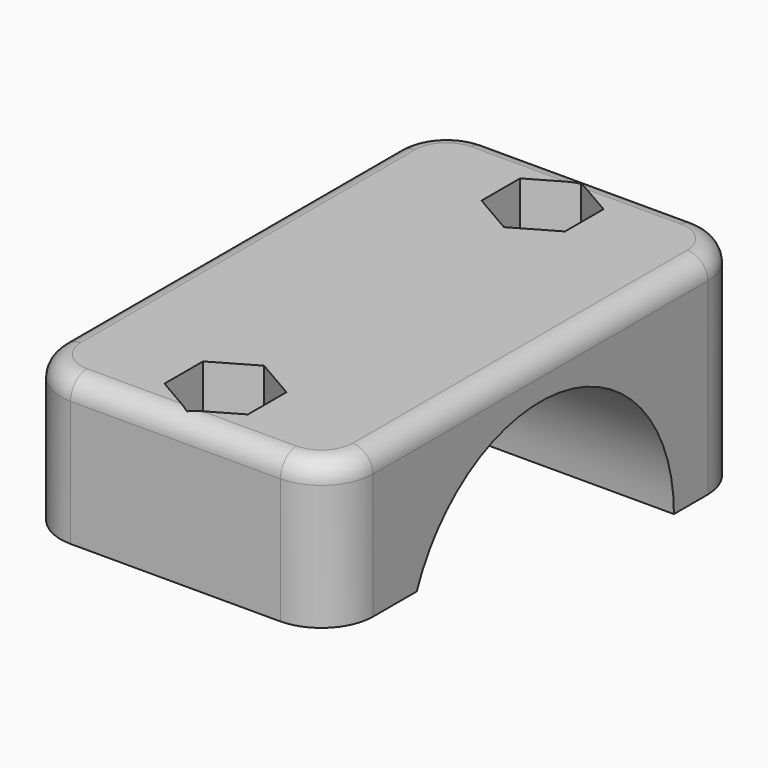
from build123d import *

# Parameters (mm, degrees)
F0_W         = 30
F0_H         = 25
F1_DEPTH     = 20
F3_DEPTH     = 50
F4_D         = 5
F5_R         = 2.5
F6_DEPTH     = 6
F7_T1_DEPTH  = 45.0048285071
F8_T1_DEPTH  = 40.1245744794
F8_T3_DEPTH  = 20.1245744794
F8_T6_ANGLE  = 88.5507069449
F8_T8_ANGLE  = 88.5507069449
F8_T10_ANGLE = 88.550706945
F8_T12_ANGLE = 88.550706945
F9_W         = 14.9377127603
F9_H         = 6
F10_DEPTH    = 50


# Not quite as in the source:
# - a fillet or chamfer that OpenCascade refuses, or shapes differently, is made with other operations: its cross-section is extruded or revolved along the edge and cut away or added


with BuildPart() as f1:
    # F0 (on Top) → F1 (new body)
    with BuildSketch(Plane.XY):
        with Locations((0, 12.5)):
            Rectangle(F0_W, F0_H)
        with Locations((0, -12.5)):
            Rectangle(F0_W, F0_H)
    extrude(amount=F1_DEPTH)

    # F2 (on face) → F3 (cut)
    with BuildSketch(Plane.YZ.offset(15)):
        with BuildLine():
            Line((-16, 0), (16, 0))
            ThreePointArc((16, 0), (0, 16), (-16, 0))
        make_face()
        with BuildLine():
            ThreePointArc((-16, 0), (0, -16), (16, 0))
            Line((16, 0), (-16, 0))
        make_face()
    extrude(amount=-F3_DEPTH, mode=Mode.SUBTRACT)

    # F4 (through all)
    with Locations(Plane(origin=(0, 0, 0), x_dir=(1, 0, 0), z_dir=(0, 0, -1))):
        with Locations((0, -19), (0, 19)):
            Hole(F4_D / 2)

    # F5 (on face) → F6 (cut)
    with BuildSketch(Plane.XY.offset(20)):
        Polygon((4, 16.6905989232), (4, 21.3094010768), (0, 23.6188021535), (-4, 21.3094010768), (-4, 16.6905989232), (0, 14.3811978465), align=None)
        with Locations((0, 19)):
            Circle(F5_R, mode=Mode.SUBTRACT)
        Polygon((4, -21.3094010768), (4, -16.6905989232), (0, -14.3811978465), (-4, -16.6905989232), (-4, -21.3094010768), (0, -23.6188021535), align=None)
        with Locations((0, -19)):
            Circle(F5_R, mode=Mode.SUBTRACT)
    extrude(amount=-F6_DEPTH, mode=Mode.SUBTRACT)

    # F7: fillet of radius 5 on 4 edges, made by hand

    # F7_s2 → F7_t1 (cut)
    with BuildSketch(Plane.XY.offset(-12.5024142536)):
        with BuildLine():
            ThreePointArc((-15.0004, 19.9990343146), (-13.5355339059, 23.5355339059), (-9.9990343146, 25.0004))
            Line((-9.9990343146, 25.0004), (-9.9990343146, 25.5005365685))
            ThreePointArc((-9.9990343146, 25.5005365685), (-12.4995171573, 25.5001365685), (-15, 25.5001365685))
            Line((-15, 25.5001365685), (-15.5001365685, 25))
            ThreePointArc((-15.5001365685, 25), (-15.5001365685, 22.4995171573), (-15.5005365685, 19.9990343146))
            Line((-15.5005365685, 19.9990343146), (-15.0004, 19.9990343146))
        make_face()
        with BuildLine():
            ThreePointArc((9.9990343146, 25.0004), (13.5355339059, 23.5355339059), (15.0004, 19.9990343146))
            Line((15.0004, 19.9990343146), (15.5005365685, 19.9990343146))
            ThreePointArc((15.5005365685, 19.9990343146), (15.5001365685, 22.4995171573), (15.5001365685, 25))
            Line((15.5001365685, 25), (15, 25.5001365685))
            ThreePointArc((15, 25.5001365685), (12.4995171573, 25.5001365685), (9.9990343146, 25.5005365685))
            Line((9.9990343146, 25.5005365685), (9.9990343146, 25.0004))
        make_face()
        with BuildLine():
            ThreePointArc((-15.0004, -19.9990343146), (-13.5355339059, -23.5355339059), (-9.9990343146, -25.0004))
            Line((-9.9990343146, -25.0004), (-9.9990343146, -25.5005365685))
            ThreePointArc((-9.9990343146, -25.5005365685), (-12.4995171573, -25.5001365685), (-15, -25.5001365685))
            Line((-15, -25.5001365685), (-15.5001365685, -25))
            ThreePointArc((-15.5001365685, -25), (-15.5001365685, -22.4995171573), (-15.5005365685, -19.9990343146))
            Line((-15.5005365685, -19.9990343146), (-15.0004, -19.9990343146))
        make_face()
        with BuildLine():
            ThreePointArc((9.9990343146, -25.0004), (13.5355339059, -23.5355339059), (15.0004, -19.9990343146))
            Line((15.0004, -19.9990343146), (15.5005365685, -19.9990343146))
            ThreePointArc((15.5005365685, -19.9990343146), (15.5001365685, -22.4995171573), (15.5001365685, -25))
            Line((15.5001365685, -25), (15, -25.5001365685))
            ThreePointArc((15, -25.5001365685), (12.4995171573, -25.5001365685), (9.9990343146, -25.5005365685))
            Line((9.9990343146, -25.5005365685), (9.9990343146, -25.0004))
        make_face()
    extrude(amount=F7_T1_DEPTH, mode=Mode.SUBTRACT)

    # F8: fillet of radius 2 on 8 edges, made by hand

    # F8_s2 → F8_t1 (cut)
    with BuildSketch(Plane.XZ.offset(-20.0622872397)):
        with BuildLine():
            ThreePointArc((12.9990343146, 20.0004), (14.4142135624, 19.4142135624), (15.0004, 17.9990343146))
            Line((15.0004, 17.9990343146), (15.2005365685, 17.9990343146))
            ThreePointArc((15.2005365685, 17.9990343146), (15.2001365685, 18.9995171573), (15.2001365685, 20))
            Line((15.2001365685, 20), (15, 20.2001365685))
            ThreePointArc((15, 20.2001365685), (13.9995171573, 20.2001365685), (12.9990343146, 20.2005365685))
            Line((12.9990343146, 20.2005365685), (12.9990343146, 20.0004))
        make_face()
        with BuildLine():
            ThreePointArc((-15.0004, 17.9990343146), (-14.4142135624, 19.4142135624), (-12.9990343146, 20.0004))
            Line((-12.9990343146, 20.0004), (-12.9990343146, 20.2005365685))
            ThreePointArc((-12.9990343146, 20.2005365685), (-13.9995171573, 20.2001365685), (-15, 20.2001365685))
            Line((-15, 20.2001365685), (-15.2001365685, 20))
            ThreePointArc((-15.2001365685, 20), (-15.2001365685, 18.9995171573), (-15.2005365685, 17.9990343146))
            Line((-15.2005365685, 17.9990343146), (-15.0004, 17.9990343146))
        make_face()
    extrude(amount=F8_T1_DEPTH, mode=Mode.SUBTRACT)

    # F8_s4 → F8_t3 (cut)
    with BuildSketch(Plane.YZ.offset(-10.0622872397)):
        with BuildLine():
            ThreePointArc((22.9990343146, 20.0004), (24.4142135624, 19.4142135624), (25.0004, 17.9990343146))
            Line((25.0004, 17.9990343146), (25.2005365685, 17.9990343146))
            ThreePointArc((25.2005365685, 17.9990343146), (25.2001365685, 18.9995171573), (25.2001365685, 20))
            Line((25.2001365685, 20), (25, 20.2001365685))
            ThreePointArc((25, 20.2001365685), (23.9995171573, 20.2001365685), (22.9990343146, 20.2005365685))
            Line((22.9990343146, 20.2005365685), (22.9990343146, 20.0004))
        make_face()
        with BuildLine():
            ThreePointArc((-22.9990343146, 20.0004), (-24.4142135624, 19.4142135624), (-25.0004, 17.9990343146))
            Line((-25.0004, 17.9990343146), (-25.2005365685, 17.9990343146))
            ThreePointArc((-25.2005365685, 17.9990343146), (-25.2001365685, 18.9995171573), (-25.2001365685, 20))
            Line((-25.2001365685, 20), (-25, 20.2001365685))
            ThreePointArc((-25, 20.2001365685), (-23.9995171573, 20.2001365685), (-22.9990343146, 20.2005365685))
            Line((-22.9990343146, 20.2005365685), (-22.9990343146, 20.0004))
        make_face()
    extrude(amount=F8_T3_DEPTH, mode=Mode.SUBTRACT)

    # F8_s5 → F8_t6 (revolve, cut)
    with BuildSketch(Plane(origin=(-9.744524799, 0.1232501355, 0), x_dir=(0, 0, 1), z_dir=(0.9999200218, -0.0126471306, 0))):
        with BuildLine():
            ThreePointArc((17.9990343146, 25.1256596074), (19.4142135624, 24.5394731698), (20.0004, 23.124293922))
            Line((20.0004, 23.124293922), (20.2005365685, 23.124293922))
            ThreePointArc((20.2005365685, 23.124293922), (20.2001365685, 24.1247767647), (20.2001365685, 25.1252596074))
            Line((20.2001365685, 25.1252596074), (20, 25.325396176))
            ThreePointArc((20, 25.325396176), (18.9995171573, 25.325396176), (17.9990343146, 25.325796176))
            Line((17.9990343146, 25.325796176), (17.9990343146, 25.1256596074))
        make_face()
    revolve(axis=Axis((-9.9990343145, -19.9990343145, 20), (0, 0, -1)), revolution_arc=F8_T6_ANGLE, mode=Mode.SUBTRACT)

    # F8_s7 → F8_t8 (revolve, cut)
    with BuildSketch(Plane(origin=(0.2513108261, 19.8693864913, 0), x_dir=(0, 0, 1), z_dir=(-0.0126471306, -0.9999200218, 0))):
        with BuildLine():
            ThreePointArc((20.0004, 13.25156501), (19.4142135624, 14.6667442578), (17.9990343146, 15.2529306954))
            Line((17.9990343146, 15.2529306954), (17.9990343146, 15.4530672639))
            ThreePointArc((17.9990343146, 15.4530672639), (18.9995171573, 15.4526672639), (20, 15.4526672639))
            Line((20, 15.4526672639), (20.2001365685, 15.2525306954))
            ThreePointArc((20.2001365685, 15.2525306954), (20.2001365685, 14.2520478527), (20.2005365685, 13.25156501))
            Line((20.2005365685, 13.25156501), (20.0004, 13.25156501))
        make_face()
    revolve(axis=Axis((-9.9990343145, 19.9990343145, 20), (0, 0, -1)), revolution_arc=F8_T8_ANGLE, mode=Mode.SUBTRACT)

    # F8_s9 → F8_t10 (revolve, cut)
    with BuildSketch(Plane(origin=(9.744524799, -0.1232501355, 0), x_dir=(0, 0, 1), z_dir=(-0.9999200218, 0.0126471306, 0))):
        with BuildLine():
            ThreePointArc((20.0004, 23.124293922), (19.4142135624, 24.5394731698), (17.9990343146, 25.1256596074))
            Line((17.9990343146, 25.1256596074), (17.9990343146, 25.325796176))
            ThreePointArc((17.9990343146, 25.325796176), (18.9995171573, 25.325396176), (20, 25.325396176))
            Line((20, 25.325396176), (20.2001365685, 25.1252596074))
            ThreePointArc((20.2001365685, 25.1252596074), (20.2001365685, 24.1247767647), (20.2005365685, 23.124293922))
            Line((20.2005365685, 23.124293922), (20.0004, 23.124293922))
        make_face()
    revolve(axis=Axis((9.9990343145, 19.9990343145, 20), (0, 0, -1)), revolution_arc=F8_T10_ANGLE, mode=Mode.SUBTRACT)

    # F8_s11 → F8_t12 (revolve, cut)
    with BuildSketch(Plane(origin=(-0.2513108261, -19.8693864913, 0), x_dir=(0, 0, 1), z_dir=(0.0126471306, 0.9999200218, 0))):
        with BuildLine():
            ThreePointArc((20.0004, 13.25156501), (19.4142135624, 14.6667442578), (17.9990343146, 15.2529306954))
            Line((17.9990343146, 15.2529306954), (17.9990343146, 15.4530672639))
            ThreePointArc((17.9990343146, 15.4530672639), (18.9995171573, 15.4526672639), (20, 15.4526672639))
            Line((20, 15.4526672639), (20.2001365685, 15.2525306954))
            ThreePointArc((20.2001365685, 15.2525306954), (20.2001365685, 14.2520478527), (20.2005365685, 13.25156501))
            Line((20.2005365685, 13.25156501), (20.0004, 13.25156501))
        make_face()
    revolve(axis=Axis((9.9990343145, -19.9990343145, 20), (0, 0, -1)), revolution_arc=F8_T12_ANGLE, mode=Mode.SUBTRACT)

    # F9 (on face) → F10 (cut)
    with BuildSketch(Plane.YZ.offset(15)):
        with BuildLine():
            Line((-16, 0), (0, 0))
            Line((0, 0), (0, 6))
            Line((0, 6), (-14.8323969742, 6))
            ThreePointArc((-14.8323969742, 6), (-15.70538684, 3.0562761993), (-16, 0))
        make_face()
        with BuildLine():
            Line((-20.0622872397, 0), (-16, 0))
            ThreePointArc((-16, 0), (-15.70538684, 3.0562761993), (-14.8323969742, 6))
            Line((-14.8323969742, 6), (-20.0622872397, 6))
            Line((-20.0622872397, 6), (-20.0622872397, 0))
        make_face()
        with Locations((-27.5311436198, 3)):
            Rectangle(F9_W, F9_H)
    extrude(amount=-F10_DEPTH, mode=Mode.SUBTRACT)


solid = f1.part
